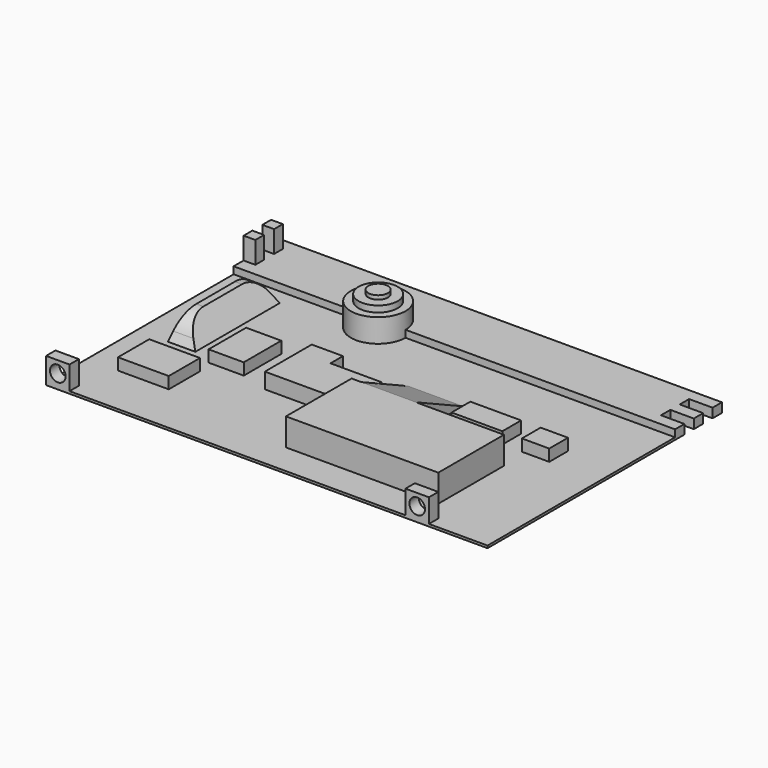
from build123d import *

# Parameters (mm, degrees)
F0_W         = 113
F0_H         = 75
F1_DEPTH     = 0.6
F2_W         = 113
F2_H         = 15
F3_DEPTH     = 1.8
F4_R         = 7
F5_DEPTH     = 6
F6_R         = 5
F7_DEPTH     = 1.6
F8_R         = 2.5
F9_DEPTH     = 1
F10_W        = 13
F10_H        = 10
F10_W_2      = 9
F10_H_2      = 12
F10_H_3      = 6
F10_W_3      = 7
F11_DEPTH    = 3
F13_W        = 39
F13_H        = 21
F14_DEPTH    = 7
F15_DEPTH    = 4
F18_DEPTH    = 14
F19_W        = 7
F19_H        = 27
F21_W        = 1.8
F21_H        = 21
F23_T1_DEPTH = 23.4311896062
F23_T6_DEPTH = 23.4311896062
F24_W        = 3
F24_H        = 2.8
F25_DEPTH    = 5.6
F26_W        = 6
F26_H        = 3
F27_DEPTH    = 3
F28_W        = 6
F28_H        = 3
F29_DEPTH    = 6
F30_R        = 2
F31_DEPTH    = 4


# Not quite as in the source:
# - a fillet or chamfer that OpenCascade refuses, or shapes differently, is made with other operations: its cross-section is extruded or revolved along the edge and cut away or added


with BuildPart() as f1:
    # F0 (on Top) → F1 (new body)
    with BuildSketch(Plane.XY):
        with Locations((0, 37.5)):
            Rectangle(F0_W, F0_H)
    extrude(amount=F1_DEPTH)

    # F2 (on face) → F3 (join)
    with BuildSketch(Plane.XY.offset(0.6)):
        with Locations((0, 67.5)):
            Rectangle(F2_W, F2_H)
    extrude(amount=F3_DEPTH)

    # F4 (on face) → F5 (join)
    with BuildSketch(Plane.XY.offset(0.6)):
        with Locations((-19.5, 60)):
            Circle(F4_R)
    extrude(amount=F5_DEPTH)

    # F6 (on face) → F7 (join)
    with BuildSketch(Plane.XY.offset(6.6)):
        with Locations((-19.5, 60)):
            Circle(F6_R)
    extrude(amount=F7_DEPTH)

    # F8 (on face) → F9 (join)
    with BuildSketch(Plane.XY.offset(8.2)):
        with Locations((-19.5, 60)):
            Circle(F8_R)
    extrude(amount=F9_DEPTH)

    # F10 (on face) → F11 (join)
    with BuildSketch(Plane.XY.offset(0.6)):
        with Locations((-42, 18)):
            Rectangle(F10_W, F10_H)
        with Locations((-32, 33)):
            Rectangle(F10_W_2, F10_H_2)
        with Locations((25, 39)):
            Rectangle(F10_W, F10_H_3)
        with Locations((40, 39)):
            Rectangle(F10_W_3, F10_H_3)
    extrude(amount=F11_DEPTH)

    # F13 (on face) → F14 (join)
    with BuildSketch(Plane.XY.offset(0.6)):
        with Locations((18, 18.5)):
            Rectangle(F13_W, F13_H)
    extrude(amount=F14_DEPTH)

    # F12 (on face) → F15 (join)
    with BuildSketch(Plane.XY.offset(0.6)):
        Polygon((-12.5, 40), (-20.5, 40), (-20.5, 25), (0.5, 25), (0.5, 36), (-12.5, 36), align=None)
    extrude(amount=F15_DEPTH)

    # F17 (on offset) → F18 (join)
    with BuildSketch(Plane.YZ.offset(15)):
        Polygon((29, 0.6), (44, 0.6), (29, 7.6), align=None)
    extrude(amount=-F18_DEPTH)

    # F19 (on face) → F22 section 0
    with BuildSketch(Plane.XY.offset(0.6)):
        with Locations((-45, 42.5)):
            Rectangle(F19_W, F19_H)
    # F21 (on offset) → F22 section 1
    with BuildSketch(Plane.XY.offset(6.6)):
        with Locations((-46.2, 42.5)):
            Rectangle(F21_W, F21_H)
    loft()

    # F23: fillet of radius 7 on 2 edges, made by hand

    # F23_s2 → F23_t1 (cut)
    with BuildSketch(Plane.YZ.offset(-57.9155948031)):
        with BuildLine():
            ThreePointArc((54.9347524158, 2.7304951685), (52.3538798636, 5.5545556585), (48.6737620788, 6.6))
            Line((48.6737620788, 6.6), (53, 6.6))
            Line((53, 6.6), (54.9347524158, 2.7304951685))
        make_face()
    extrude(amount=F23_T1_DEPTH, mode=Mode.SUBTRACT)


with BuildPart() as f23_tool4:
    # F23_s5 → F23_t6 (new body)
    with BuildSketch(Plane.YZ.offset(-57.9155948031)):
        with BuildLine():
            ThreePointArc((30.0652475842, 2.7304951685), (32.6461201364, 5.5545556585), (36.3262379212, 6.6))
            Line((36.3262379212, 6.6), (32, 6.6))
            Line((32, 6.6), (30.0652475842, 2.7304951685))
        make_face()
    extrude(amount=F23_T6_DEPTH)

    split(bisect_by=Plane.YZ.offset(-36.5), keep=Keep.BOTTOM)


with BuildPart() as f1_1:
    add(f1.part)

    # F23_t3: cut F23_tool4
    add(f23_tool4.part, mode=Mode.SUBTRACT)

    # F24 (on face) → F25 (join)
    with BuildSketch(Plane.XY.offset(2.4)):
        with Locations((-55, 70.6)):
            Rectangle(F24_W, F24_H)
        with Locations((-55, 64.6)):
            Rectangle(F24_W, F24_H)
    extrude(amount=F25_DEPTH)

    # F26 (on face) → F27 (cut)
    with BuildSketch(Plane.XY.offset(2.4)):
        with Locations((53.5, 70.5)):
            Rectangle(F26_W, F26_H)
        with Locations((53.5, 64.5)):
            Rectangle(F26_W, F26_H)
    extrude(amount=-F27_DEPTH, mode=Mode.SUBTRACT)

    # F28 (on face) → F29 (join)
    with BuildSketch(Plane.XY.offset(0.6)):
        with Locations((-53.5, 1.5)):
            Rectangle(F28_W, F28_H)
        with Locations((38.5, 1.5)):
            Rectangle(F28_W, F28_H)
    extrude(amount=F29_DEPTH)

    # F30 (on face) → F31 (cut)
    with BuildSketch(Plane.XZ):
        with Locations((-53.5, 3.6)):
            Circle(F30_R)
        with Locations((38.5, 3.6)):
            Circle(F30_R)
    extrude(amount=-F31_DEPTH, mode=Mode.SUBTRACT)


solid = f1_1.part
